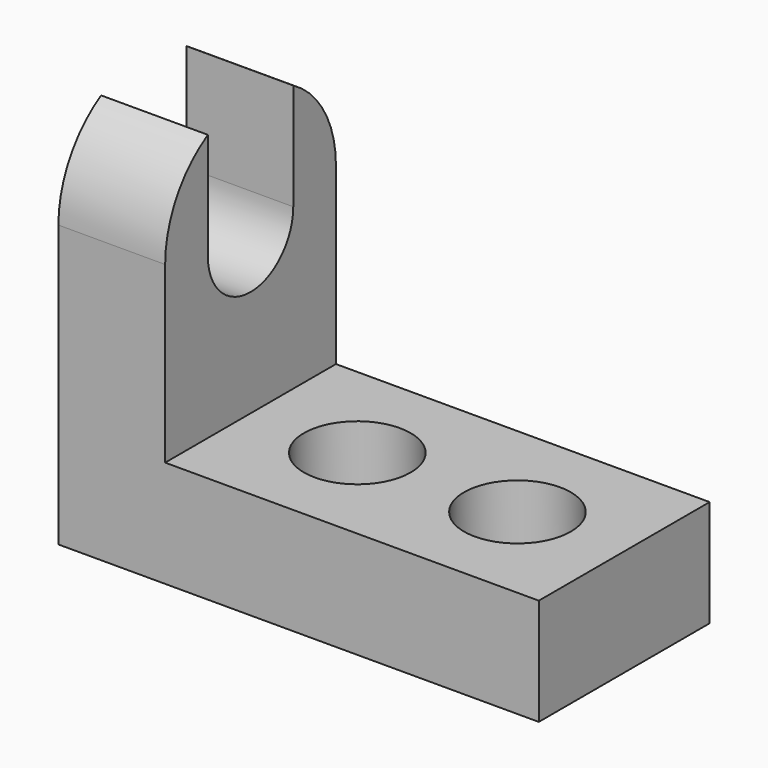
from build123d import *

# Parameters (mm, degrees)
F0_W        = 57.15
F0_H        = 44.45
F1_DEPTH    = 25.4
F2_W        = 44.45
F2_H        = 31.75
F3_DEPTH    = 25.4
F4_R        = 6.35
F5_DEPTH    = 25.4
F7_DEPTH    = 25.4
F8_T1_DEPTH = 67.6926131403


# Not quite as in the source:
# - a fillet or chamfer that OpenCascade refuses, or shapes differently, is made with other operations: its cross-section is extruded or revolved along the edge and cut away or added


with BuildPart() as f1:
    # F0 (on Front) → F1 (new body)
    with BuildSketch(Plane.XZ):
        with Locations((28.575, 22.225)):
            Rectangle(F0_W, F0_H)
    extrude(amount=F1_DEPTH)

    # F2 (on face) → F3 (cut)
    with BuildSketch(Plane.XZ.offset(25.4)):
        with Locations((34.925, 28.575)):
            Rectangle(F2_W, F2_H)
    extrude(amount=-F3_DEPTH, mode=Mode.SUBTRACT)

    # F4 (on face) → F5 (cut)
    with BuildSketch(Plane.XY.offset(12.7)):
        with Locations((25.4, -12.7)):
            Circle(F4_R)
        with Locations((44.45, -12.7)):
            Circle(F4_R)
    extrude(amount=-F5_DEPTH, mode=Mode.SUBTRACT)

    # F6 (on face) → F7 (cut)
    with BuildSketch(Plane.YZ.offset(12.7)):
        with BuildLine():
            ThreePointArc((-19.05, 31.75), (-12.7, 38.1), (-6.35, 31.75))
            Line((-6.35, 31.75), (-6.35, 44.45))
            Line((-6.35, 44.45), (-19.05, 44.45))
            Line((-19.05, 44.45), (-19.05, 31.75))
        make_face()
        with BuildLine():
            ThreePointArc((-19.05, 31.75), (-12.7, 25.4), (-6.35, 31.75))
            ThreePointArc((-6.35, 31.75), (-12.7, 38.1), (-19.05, 31.75))
        make_face()
    extrude(amount=-F7_DEPTH, mode=Mode.SUBTRACT)

    # F8: fillet of radius 12.7 on 2 edges, made by hand

    # F8_s2 → F8_t1 (cut)
    with BuildSketch(Plane.YZ.offset(-27.4963065702)):
        with BuildLine():
            ThreePointArc((-25.4, 33.4514773719), (-23.6985226281, 39.8014773719), (-19.05, 44.45))
            Line((-19.05, 44.45), (-25.4, 44.45))
            Line((-25.4, 44.45), (-25.4, 33.4514773719))
        make_face()
        with BuildLine():
            ThreePointArc((0, 33.4514773719), (-1.7014773719, 39.8014773719), (-6.35, 44.45))
            Line((-6.35, 44.45), (0, 44.45))
            Line((0, 44.45), (0, 33.4514773719))
        make_face()
    extrude(amount=F8_T1_DEPTH, mode=Mode.SUBTRACT)


solid = f1.part
